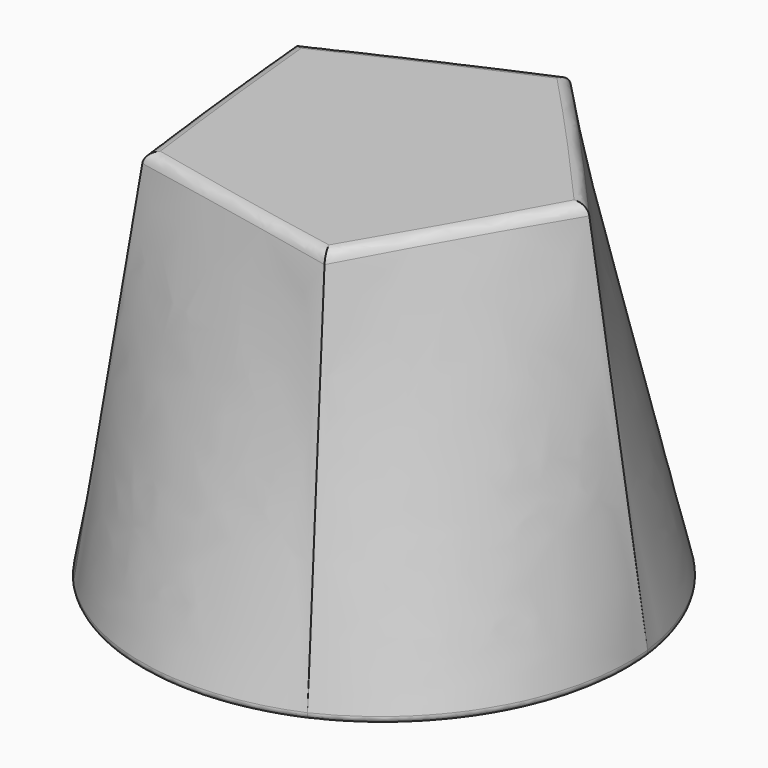
from build123d import *

# Parameters (mm, degrees)
F4_R = 2
F5_R = 1


# Not quite as in the source:
# - the arcs of a loft's sections are written as splines that run evenly, so that the points pair up as in the source's solid


with BuildPart() as f3:
    # F2 (on offset) → F3 section 0
    with BuildSketch(Plane.XY.offset(66.1)):
        Polygon((6.5035684594, 31.6557302665), (-28.09667537, 15.9674197842), (-23.8682688089, -21.7873221272), (13.3452739935, -29.4327253826), (32.116101726, 3.5968974592), align=None)
    # F1 (on Top) → F3 section 1
    with BuildSketch(Plane.XY):
        with BuildLine():
            add(Edge.make_bspline(
                [(8.4533662401, 41.1462542772), (6.2989534041, 41.5888714985), (4.109728025, 41.861929985), (-0.2845300293, 42.0622168837), (-2.4895181694, 41.989443266), (-6.8610073891, 41.4998508927), (-9.0274641643, 41.0830370989), (-13.2685439766, 39.9156208426), (-15.343124031, 39.1650302116), (-19.3493649757, 37.348535735), (-21.2809852632, 36.2826502992), (-24.9537403921, 33.8618057249), (-26.6948380106, 32.5068711213), (-29.9436719034, 29.541285677), (-31.4513752512, 27.9306648922), (-34.1962908351, 24.4933611338), (-35.4334752519, 22.6667129969), (-36.5201794236, 20.7545208738)],
                knots=[0, 0, 0, 0, 0.125, 0.125, 0.25, 0.25, 0.375, 0.375, 0.5, 0.5, 0.625, 0.625, 0.75, 0.75, 0.875, 0.875, 1, 1, 1, 1], degree=3))
            add(Edge.make_bspline(
                [(-36.5201794236, 20.7545208738), (-37.6068835954, 18.8423287507), (-38.5430854949, 16.8446314011), (-40.0914700715, 12.7273356997), (-40.7036370559, 10.6077790761), (-41.5888714985, 6.2989534041), (-41.861929985, 4.109728025), (-42.0622168837, -0.2845300293), (-41.989443266, -2.4895181694), (-41.4998508927, -6.8610073891), (-41.0830370989, -9.0274641643), (-39.9156208426, -13.2685439766), (-39.1650302116, -15.343124031), (-37.348535735, -19.3493649757), (-36.2826502992, -21.2809852632), (-33.8618057249, -24.9537403921), (-32.5068711213, -26.6948380106), (-31.0240783991, -28.319254957)],
                knots=[0, 0, 0, 0, 0.125, 0.125, 0.25, 0.25, 0.375, 0.375, 0.5, 0.5, 0.625, 0.625, 0.75, 0.75, 0.875, 0.875, 1, 1, 1, 1], degree=3))
            add(Edge.make_bspline(
                [(-31.0240783991, -28.319254957), (-29.541285677, -29.9436719034), (-27.9306648922, -31.4513752512), (-24.4933611338, -34.1962908351), (-22.6667129969, -35.4334752519), (-18.8423287507, -37.6068835954), (-16.8446314011, -38.5430854949), (-12.7273356997, -40.0914700715), (-10.6077790761, -40.7036370559), (-6.2989534041, -41.5888714985), (-4.109728025, -41.861929985), (0.2845300293, -42.0622168837), (2.4895181694, -41.989443266), (6.8610073891, -41.4998508927), (9.0274641643, -41.0830370989), (13.2685439766, -39.9156208426), (15.343124031, -39.1650302116), (17.3462445033, -38.2567829733)],
                knots=[0, 0, 0, 0, 0.125, 0.125, 0.25, 0.25, 0.375, 0.375, 0.5, 0.5, 0.625, 0.625, 0.75, 0.75, 0.875, 0.875, 1, 1, 1, 1], degree=3))
            add(Edge.make_bspline(
                [(17.3462445033, -38.2567829733), (19.3493649757, -37.348535735), (21.2809852632, -36.2826502992), (24.9537403921, -33.8618057249), (26.6948380106, -32.5068711213), (29.9436719034, -29.541285677), (31.4513752512, -27.9306648922), (34.1962908351, -24.4933611338), (35.4334752519, -22.6667129969), (37.6068835954, -18.8423287507), (38.5430854949, -16.8446314011), (40.0914700715, -12.7273356997), (40.7036370559, -10.6077790761), (41.5888714985, -6.2989534041), (41.861929985, -4.109728025), (42.0622168837, 0.2845300293), (41.989443266, 2.4895181694), (41.7446470794, 4.6752627793)],
                knots=[0, 0, 0, 0, 0.125, 0.125, 0.25, 0.25, 0.375, 0.375, 0.5, 0.5, 0.625, 0.625, 0.75, 0.75, 0.875, 0.875, 1, 1, 1, 1], degree=3))
            add(Edge.make_bspline(
                [(41.7446470794, 4.6752627793), (41.4998508927, 6.8610073891), (41.0830370989, 9.0274641643), (39.9156208426, 13.2685439766), (39.1650302116, 15.343124031), (37.348535735, 19.3493649757), (36.2826502992, 21.2809852632), (33.8618057249, 24.9537403921), (32.5068711213, 26.6948380106), (29.541285677, 29.9436719034), (27.9306648922, 31.4513752512), (24.4933611338, 34.1962908351), (22.6667129969, 35.4334752519), (18.8423287507, 37.6068835954), (16.8446314011, 38.5430854949), (12.7273356997, 40.0914700715), (10.6077790761, 40.7036370559), (8.4533662401, 41.1462542772)],
                knots=[0, 0, 0, 0, 0.125, 0.125, 0.25, 0.25, 0.375, 0.375, 0.5, 0.5, 0.625, 0.625, 0.75, 0.75, 0.875, 0.875, 1, 1, 1, 1], degree=3))
        make_face()
    loft(ruled=True)

    # F4
    f4_edges = [f3.edges().sort_by_distance(p)[0] for p in [
        (22.730688, -12.917914, 66.1),
        (19.309835, 17.626314, 66.1),
        (-10.796553, 23.811575, 66.1),
        (-25.982472, -2.909951, 66.1),
        (-5.261497, -25.610024, 66.1),
    ]]
    fillet(f4_edges, radius=F4_R)

    # F5
    f5_edges = [f3.edges().sort_by_distance(p)[0] for p in [
        (36.520179, -20.754521, 0),
        (31.024078, 28.319255, 0),
        (-17.346245, 38.256783, 0),
        (-41.744647, -4.675263, 0),
        (-8.453366, -41.146254, 0),
    ]]
    fillet(f5_edges, radius=F5_R)


solid = f3.part
